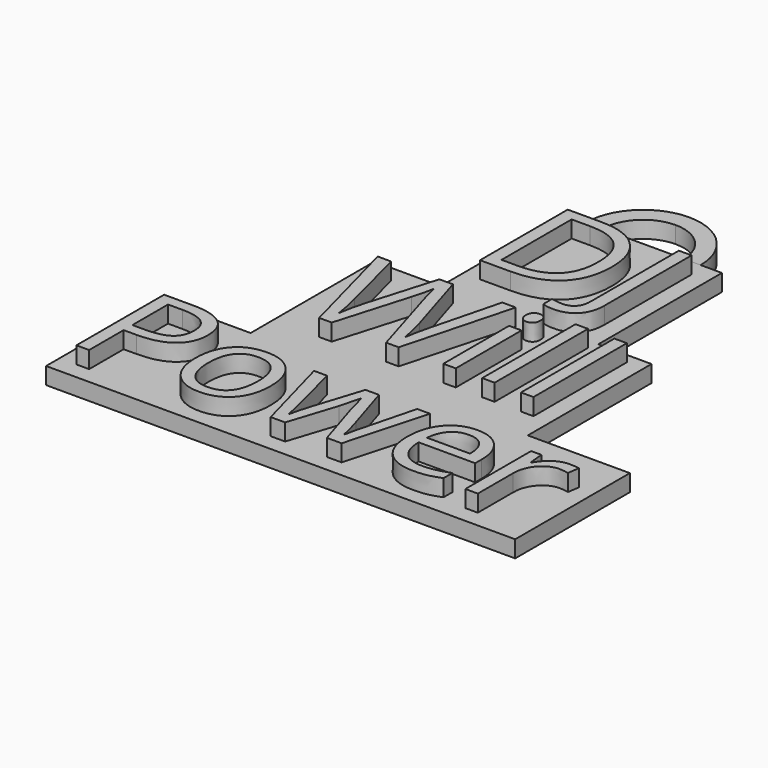
from build123d import *

# Parameters (mm, degrees)
F0_TEXT_SIZE = 28.9480453307
F1_DEPTH     = 3.175
F2_W         = 29.7029309441
F2_H         = 29.1483926381
F3_DEPTH     = 3.175
F5_DEPTH     = 3.175


# Not quite as in the source:
# - Text() gives the source's letters only with a copy of the font that has no kerning and outlines rounded to 1/6400 em; it was checked with that copy


with BuildPart() as f1:
    # F0 (on Top) → F1 (new body)
    with BuildSketch(Plane.XY):
        with Locations((-16.3872292965, 24.3745971898)):
            Text('DJ', F0_TEXT_SIZE, font='Open Sans', text_align=(TextAlign.LEFT, TextAlign.BOTTOM))
        with Locations((-26.4308440866, -4.7737954483)):
            Text('Will', F0_TEXT_SIZE, font='Open Sans', text_align=(TextAlign.LEFT, TextAlign.BOTTOM))
        with Locations((-45.8305575903, -33.9221880863)):
            Text('Power', F0_TEXT_SIZE, font='Open Sans', text_align=(TextAlign.LEFT, TextAlign.BOTTOM))
    extrude(amount=F1_DEPTH)


with BuildPart() as f3:
    # F2 (on face) → F3 (new body)
    with BuildSketch(Plane(origin=(0, 0, 0), x_dir=(1, 0, 0), z_dir=(0, 0, -1))):
        Polygon((42.2617241345, 37.0971880863), (-46.1650306422, 37.0971880863), (-46.1650306422, 10.0809975995), (-29.2259009917, 10.0809975995), (23.0248433858, 10.0809975995), (42.2617241345, 10.0809975995), align=None)
        Polygon((23.0248433858, 10.0809975995), (-29.2259009917, 10.0809975995), (-29.2259009917, -19.0673950386), (-16.7217023484, -19.0673950386), (12.9812285957, -19.0673950386), (23.0248433858, -19.0673950386), align=None)
        with Locations((-1.8702368764, -33.6415913577)):
            Rectangle(F2_W, F2_H)
    extrude(amount=F3_DEPTH)


with BuildPart() as f5:
    # F4 (on face) → F5 (new body)
    with BuildSketch(Plane.XY):
        with BuildLine():
            ThreePointArc((8.9698911842, 48.2157876767), (5.7948911842, 55.8809157372), (-1.8702368764, 59.0559157372))
            ThreePointArc((-1.8702368764, 59.0559157372), (-9.5353649369, 55.8809157372), (-12.7103649369, 48.2157876767))
            Line((-12.7103649369, 48.2157876767), (-9.5353649369, 48.2157876767))
            ThreePointArc((-9.5353649369, 48.2157876767), (-7.2903009066, 53.635851707), (-1.8702368764, 55.8809157372))
            ThreePointArc((-1.8702368764, 55.8809157372), (3.5498271539, 53.635851707), (5.7948911842, 48.2157876767))
            Line((5.7948911842, 48.2157876767), (8.9698911842, 48.2157876767))
        make_face()
    extrude(amount=-F5_DEPTH)


solid = Compound([f1.part, f3.part, f5.part])
